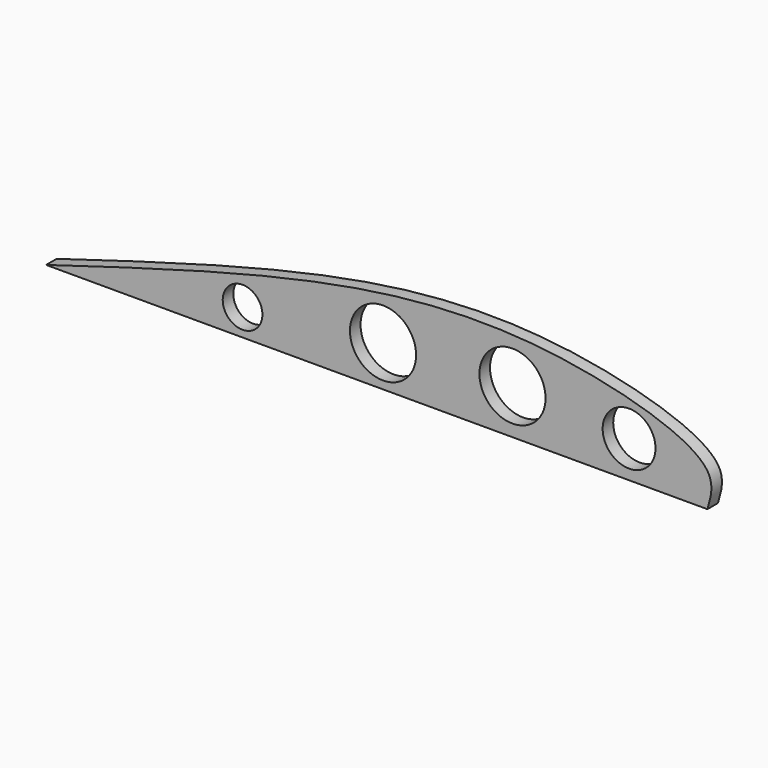
from build123d import *

# Parameters (mm, degrees)
F1_DEPTH = 1.27
F3_D     = 5.08
F4_D     = 6.35
F5_D     = 3.81


# Not quite as in the source:
# - a feature names something its author has since deleted; it is built from what else it names


with BuildPart() as f1:
    # F0 (on Front) → F1 (new body)
    with BuildSketch(Plane.XZ):
        with BuildLine():
            add(Edge.make_bspline(
                [(63.5, 0), (63.8322128437, 1.1116457049), (64.812711118, 4.3925725485), (50.520767413, 8.9452032158), (30.6942173185, 9.1884909037), (10.964974549, 3.2824308558), (0, 0)],
                knots=[0, 0, 0, 0, 0.1157736296, 0.3416959746, 0.6341325299, 1, 1, 1, 1], degree=3))
            Line((0, 0), (63.5, 0))
        make_face()
    extrude(amount=-F1_DEPTH)

    # F3 (through all)
    with Locations(Plane.XZ):
        with Locations((55.9804104269, 3.5253837705)):
            Hole(F3_D / 2)

    # F4 (through all)
    with Locations(Plane.XZ):
        with Locations((44.7878539562, 4.3252892792), (32.3550179601, 3.9246454835)):
            Hole(F4_D / 2)

    # F5 (through all)
    with Locations(Plane.XZ):
        with Locations((18.8655108213, 2.5541819632)):
            Hole(F5_D / 2)


solid = f1.part
